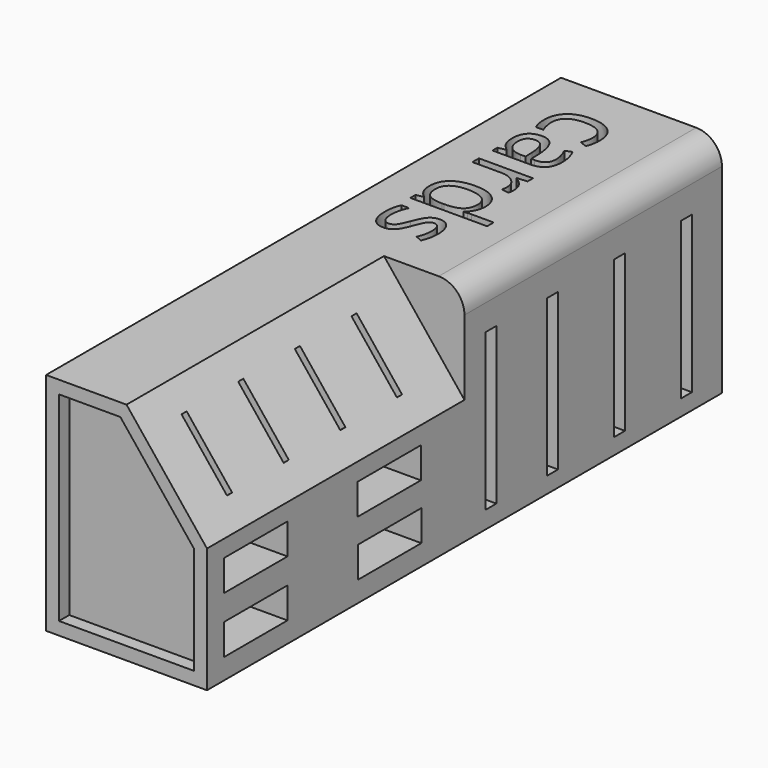
from build123d import *

# Parameters (mm, degrees)
F0_W          = 25
F0_H          = 100
F1_DEPTH      = 35
F3_DEPTH      = 50
F4_W          = 1
F4_H          = 11.3
F5_DEPTH      = 10
F6_R          = 4
F7_W          = 2.15
F7_H          = 24.3
F8_DEPTH      = 20
F7_W_2        = 12.3
F7_H_2        = 4.8
F9_DEPTH      = 12
F10_TEXT_SIZE = 15.6910818265
F11_DEPTH     = 3
F13_DEPTH     = 2


# Not quite as in the source:
# - Text() gives the source's letters only with a copy of the font that has no kerning and outlines rounded to 1/6400 em; it was checked with that copy


with BuildPart() as f1:
    # F0 (on Top) → F1 (new body)
    with BuildSketch(Plane.XY):
        Rectangle(F0_W, F0_H)
    extrude(amount=-F1_DEPTH)

    # F2 (on face) → F3 (cut)
    with BuildSketch(Plane.XZ.offset(50)):
        Polygon((12.5, 0), (0, 0), (12.5, -15.612494996), align=None)
    extrude(amount=-F3_DEPTH, mode=Mode.SUBTRACT)

    # F4 (on face) → F5 (cut)
    with BuildSketch(Plane(origin=(0, 0, 0), x_dir=(0, 1, 0), z_dir=(0.7806247498, 0, 0.625))):
        with Locations((-9.2174606398, -10)):
            Rectangle(F4_W, F4_H)
        with Locations((-20.2174606398, -10)):
            Rectangle(F4_W, F4_H)
        with Locations((-31.2174606398, -10)):
            Rectangle(F4_W, F4_H)
        with Locations((-42.2174606398, -10)):
            Rectangle(F4_W, F4_H)
    extrude(amount=-F5_DEPTH, mode=Mode.SUBTRACT)

    # F6
    f6_edges = [f1.edges().sort_by_distance(p)[0] for p in [
        (12.5, 25, 0),
    ]]
    fillet(f6_edges, radius=F6_R)

    # F7 (on face) → F8 (cut)
    with BuildSketch(Plane.YZ.offset(12.5)):
        with Locations((5.1180827379, -20.1600721195)):
            Rectangle(F7_W, F7_H)
        with Locations((17.0954090158, -20.3600721195)):
            Rectangle(F7_W, F7_H)
        with Locations((30.0954090158, -20.3600721195)):
            Rectangle(F7_W, F7_H)
        with Locations((43.0954090158, -20.3600721195)):
            Rectangle(F7_W, F7_H)
    extrude(amount=-F8_DEPTH, mode=Mode.SUBTRACT)

    # F7 (on face) → F9 (cut)
    with BuildSketch(Plane.YZ.offset(12.5)):
        with Locations((-40.5175739735, -29.4011362106)):
            Rectangle(F7_W_2, F7_H_2)
        with Locations((-14.5175739735, -29.4011362106)):
            Rectangle(F7_W_2, F7_H_2)
        with Locations((-40.5175739735, -20.6500027537)):
            Rectangle(F7_W_2, F7_H_2)
        with Locations((-14.6212725672, -20.7662601024)):
            Rectangle(F7_W_2, F7_H_2)
    extrude(amount=-F9_DEPTH, mode=Mode.SUBTRACT)

    # F10 (on face) → F11 (cut)
    with BuildSketch(Plane.XY):
        with Locations(Location((-7.0475789151, 44.7953337628), (0, 0, -90))):
            Text('cards', F10_TEXT_SIZE, font='Open Sans', text_align=(TextAlign.LEFT, TextAlign.BOTTOM))
    extrude(amount=-F11_DEPTH, mode=Mode.SUBTRACT)

    # F12 (on face) → F13 (cut)
    with BuildSketch(Plane.XZ.offset(50)):
        Polygon((10.5, -16.3144957966), (-0.9607689228, -2), (-10.5, -2), (-10.5, -33), (10.5, -33), align=None)
    extrude(amount=-F13_DEPTH, mode=Mode.SUBTRACT)


solid = f1.part
